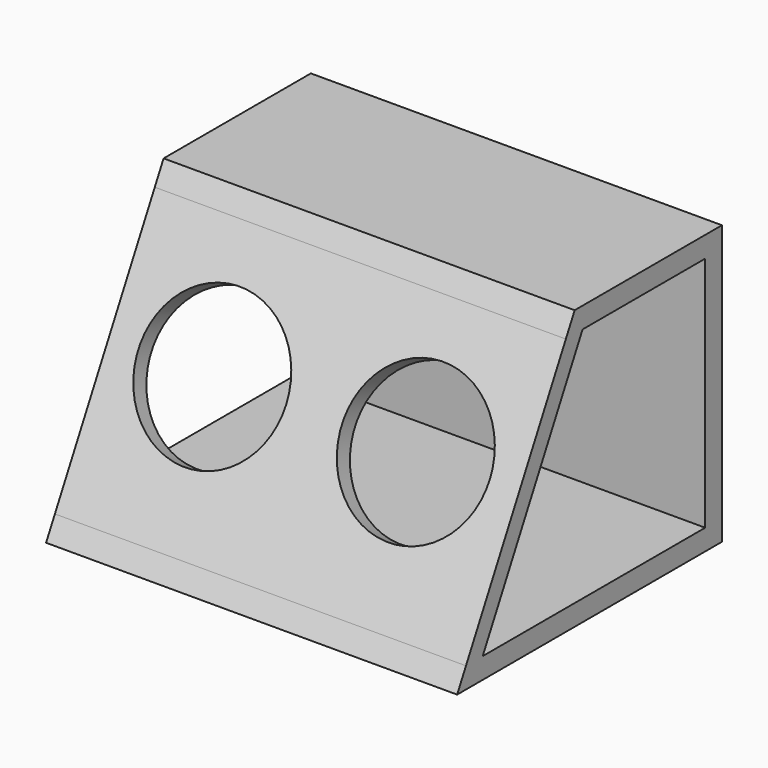
from build123d import *

# Parameters (mm, degrees)
F0_W      = 118
F0_H      = 95
F1_DEPTH  = 6
F2_W      = 118
F2_H      = 74
F3_DEPTH  = 6
F4_W      = 118
F4_H      = 6
F5_DEPTH  = 50
F7_DEPTH  = 118
F9_DEPTH  = 118.001
F11_R     = 21.25
F12_DEPTH = 5.3079525657


with BuildPart() as f1:
    # F0 (on Top) → F1 (new body)
    with BuildSketch(Plane.XY):
        Rectangle(F0_W, F0_H)
    extrude(amount=F1_DEPTH)

    # F2 (on face) → F3 (join)
    with BuildSketch(Plane(origin=(0, 47.5, 0), x_dir=(-1, 0, 0), z_dir=(0, 1, 0))):
        with Locations((0, 43)):
            Rectangle(F2_W, F2_H)
    extrude(amount=-F3_DEPTH)

    # F4 (on face) → F5 (join)
    with BuildSketch(Plane.XZ.offset(-41.5)):
        with Locations((0, 77)):
            Rectangle(F4_W, F4_H)
    extrude(amount=F5_DEPTH)

    # F6 (on face) → F7 (join)
    with BuildSketch(Plane(origin=(-59, 0, 0), x_dir=(0, -1, 0), z_dir=(-1, 0, 0))):
        Polygon((38.3378378378, 6), (44.3378378378, 6), (8.5, 74), (2.5, 74), align=None)
        Polygon((2.5, 74), (8.5, 74), (5.3378378378, 80), (-0.6621621622, 80), align=None)
        Polygon((41.5, 0), (47.5, 0), (44.3378378378, 6), (38.3378378378, 6), align=None)
    extrude(amount=-F7_DEPTH)

    # F8 (on face) → F9 (cut, through all)
    with BuildSketch(Plane.YZ.offset(59)):
        Polygon((-47.5, 6), (-47.5, 0), (-44.3378378378, 6), align=None)
        Polygon((-8.5, 80), (-8.5, 74), (-5.3378378378, 80), align=None)
    extrude(amount=-F9_DEPTH, mode=Mode.SUBTRACT)

    # F11 (on face) → F12 (cut, through all)
    with BuildSketch(Plane(origin=(0, -37.1745033586, 19.5919679863), x_dir=(1, 0, 0), z_dir=(0, -0.884658761, 0.4662390767))):
        with Locations((-29.2115788907, 25.8900932968)):
            Circle(F11_R)
        with Locations((29.2115788907, 25.8900932968)):
            Circle(F11_R)
    extrude(amount=-F12_DEPTH, mode=Mode.SUBTRACT)


solid = f1.part
